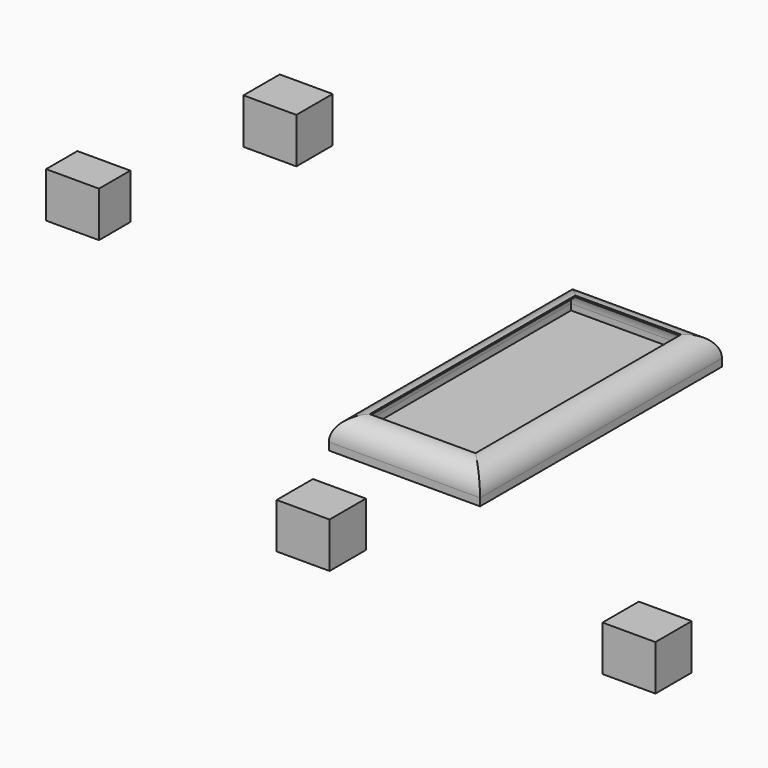
from build123d import *

# Parameters (mm, degrees)
F0_W      = 100
F0_H      = 200
F1_DEPTH  = 20
F2_R      = 15
F3_T      = -1
F4_W      = 35
F4_H      = 30
F5_DEPTH  = 30
F6_W      = 35
F6_H      = 30
F7_DEPTH  = 30
F8_W      = 35
F8_H      = 25.8680122671
F9_DEPTH  = 30
F10_W     = 35
F10_H     = 30
F11_DEPTH = 30


# Not quite as in the source:
# - a shell that OpenCascade refuses in one call is made with other operations: the cavity is built on its own and cut out


with BuildPart() as f1:
    # F0 (on Top) → F1 (new body)
    with BuildSketch(Plane.XY):
        with Locations((-239.2185236739, -96.3341407478)):
            Rectangle(F0_W, F0_H)
    extrude(amount=F1_DEPTH)

    # F2
    f2_edges = [f1.edges().sort_by_distance(p)[0] for p in [
        (-189.218524, -96.334141, 20),
        (-239.218524, -196.334141, 20),
        (-239.218524, 3.665859, 20),
        (-289.218524, -96.334141, 20),
    ]]
    fillet(f2_edges, radius=F2_R)

    # F3: a shell. OpenCascade refuses it in one call, so the cavity is built on its own and cut out:
    # the body offset inwards by the wall thickness, plus a prism from it out through each open face.
    f3_core = offset(f1.part, amount=F3_T, mode=Mode.PRIVATE)
    f3_exits = [f3_core.faces().sort_by_distance(p)[0] for p in [
        (-239.218524, -96.334141, 19),
    ]]
    add(f3_core, mode=Mode.SUBTRACT)
    extrude(f3_exits, amount=-F3_T, mode=Mode.SUBTRACT)


with BuildPart() as f5:
    # F4 (on Top) → F5 (new body)
    with BuildSketch(Plane.XY):
        with Locations((-222.2460955381, -286.3571236897)):
            Rectangle(F4_W, F4_H)
    extrude(amount=F5_DEPTH)


with BuildPart() as f7:
    # F6 (on face) → F7 (new body)
    with BuildSketch(Plane(origin=(0, -271.3571236897, 0), x_dir=(-1, 0, 0), z_dir=(0, 1, 0))):
        with Locations((30.6952949613, -6.2826325541)):
            Rectangle(F6_W, F6_H)
    extrude(amount=F7_DEPTH)


with BuildPart() as f9:
    # F8 (on Top) → F9 (new body)
    with BuildSketch(Plane.XY):
        with Locations((-546.4502573013, -73.8191474229)):
            Rectangle(F8_W, F8_H)
    extrude(amount=F9_DEPTH)


with BuildPart() as f11:
    # F10 (on Top) → F11 (new body)
    with BuildSketch(Plane.XY):
        with Locations((-518.3916091919, 56.3756684118)):
            Rectangle(F10_W, F10_H)
    extrude(amount=F11_DEPTH)


solid = Compound([f1.part, f5.part, f7.part, f9.part, f11.part])
